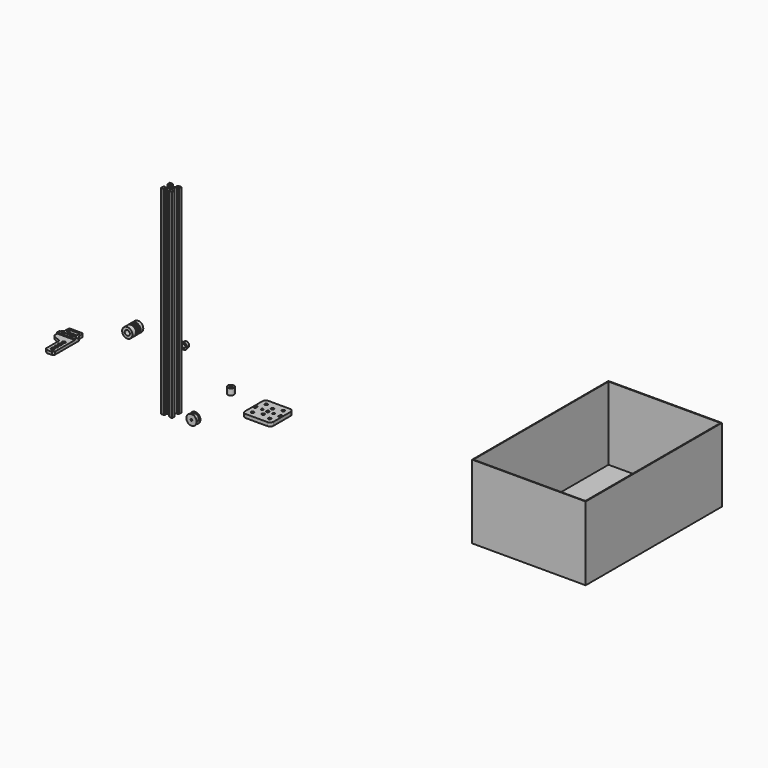
from build123d import *

# Parameters (mm, degrees)
F0_R         = 5.5
F0_R_2       = 2.5
F1_DEPTH     = 11
F2_R         = 2.51
F2_R_2       = 2
F2_W         = 2.75
F2_H         = 6.7
F3_DEPTH     = 6.35
F8_R         = 1.5
F8_R_2       = 2.15
F9_DEPTH     = 5
F10_T1_DEPTH = 20.4300979278
F10_T3_DEPTH = 14.9582429798
F11_R        = 2.1
F12_DEPTH    = 2
F14_DEPTH    = 2
F16_DEPTH    = 5
F17_SIZE     = 2
F18_W        = 199.62876
F18_H        = 299.64126
F18_W_2      = 197.0495581627
F18_H_2      = 297.1284687519
F19_DEPTH    = 129.77876
F22_DEPTH    = 350
F25_DEPTH    = 1


# Not quite as in the source:
# - a fillet or chamfer that OpenCascade refuses, or shapes differently, is made with other operations: its cross-section is extruded or revolved along the edge and cut away or added


with BuildPart() as f1:
    # F0 (on Top) → F1 (new body)
    with BuildSketch(Plane.XY):
        with Locations((46.5984568, 59.2390596867)):
            Circle(F0_R)
        with Locations((46.5984568, 59.2390596867)):
            Circle(F0_R_2, mode=Mode.SUBTRACT)
    extrude(amount=F1_DEPTH)


with BuildPart() as f3:
    # F2 (on Top) → F3 (new body)
    with BuildSketch(Plane.XY):
        with BuildLine():
            Line((145.757446865, 65.371271316), (108.097446865, 65.371271316))
            ThreePointArc((108.097446865, 65.371271316), (103.7345980251, 63.5641201559), (101.927446865, 59.201271316))
            Line((101.927446865, 59.201271316), (101.927446865, 43.721271316))
            Line((101.927446865, 43.721271316), (104.677446865, 43.721271316))
            Line((104.677446865, 43.721271316), (107.177446865, 43.721271316))
            Line((107.177446865, 43.721271316), (107.177446865, 40.371271316))
            Line((107.177446865, 40.371271316), (107.177446865, 37.021271316))
            Line((107.177446865, 37.021271316), (104.677446865, 37.021271316))
            Line((104.677446865, 37.021271316), (101.927446865, 37.021271316))
            Line((101.927446865, 37.021271316), (101.927446865, 21.541271316))
            ThreePointArc((101.927446865, 21.541271316), (103.7345980251, 17.178422476), (108.097446865, 15.371271316))
            Line((108.097446865, 15.371271316), (145.757446865, 15.371271316))
            ThreePointArc((145.757446865, 15.371271316), (150.1202957049, 17.178422476), (151.927446865, 21.541271316))
            Line((151.927446865, 21.541271316), (151.927446865, 37.021271316))
            Line((151.927446865, 37.021271316), (149.177446865, 37.021271316))
            Line((149.177446865, 37.021271316), (146.677446865, 37.021271316))
            Line((146.677446865, 37.021271316), (146.677446865, 40.371271316))
            Line((146.677446865, 40.371271316), (146.677446865, 43.721271316))
            Line((146.677446865, 43.721271316), (149.177446865, 43.721271316))
            Line((149.177446865, 43.721271316), (151.927446865, 43.721271316))
            Line((151.927446865, 43.721271316), (151.927446865, 59.201271316))
            ThreePointArc((151.927446865, 59.201271316), (150.1202957049, 63.5641201559), (145.757446865, 65.371271316))
        make_face()
        with Locations((111.927446865, 25.371271316)):
            Circle(F2_R, mode=Mode.SUBTRACT)
        with Locations((126.927446865, 30.371271316)):
            Circle(F2_R, mode=Mode.SUBTRACT)
        with Locations((116.927446865, 40.371271316)):
            Circle(F2_R_2, mode=Mode.SUBTRACT)
        with Locations((126.927446865, 40.371271316)):
            Circle(F2_R, mode=Mode.SUBTRACT)
        with Locations((141.927446865, 25.371271316)):
            Circle(F2_R, mode=Mode.SUBTRACT)
        with Locations((136.927446865, 40.371271316)):
            Circle(F2_R_2, mode=Mode.SUBTRACT)
        with Locations((126.927446865, 50.371271316)):
            Circle(F2_R, mode=Mode.SUBTRACT)
        with Locations((111.927446865, 55.371271316)):
            Circle(F2_R, mode=Mode.SUBTRACT)
        with Locations((141.927446865, 55.371271316)):
            Circle(F2_R, mode=Mode.SUBTRACT)
        Polygon((104.677446865, 43.721271316), (101.927446865, 43.721271316), (101.927446865, 40.371271316), (101.927446865, 37.021271316), (104.677446865, 37.021271316), align=None)
        with Locations((150.552446865, 40.371271316)):
            Rectangle(F2_W, F2_H)
    extrude(amount=F3_DEPTH)


with BuildPart() as f5:
    # F4 (on Top) → F5 (revolve)
    with BuildSketch(Plane.XY):
        Polygon((-173.2957138275, 117.2877326608), (-173.2957138275, 111.8661259413), (-168.7957138275, 111.8661259413), (-168.7957138275, 118.7537908554), (-172.3944602844, 117.5813526924), align=None)
        Polygon((-173.2957138275, 118.6839789152), (-173.2957138275, 117.2877326608), (-172.3944602844, 117.5813526924), (-172.3944602844, 118.9775989469), align=None)
        Polygon((-172.3944602844, 117.5813526924), (-168.7957138275, 118.7537908554), (-168.7957138275, 120.1500371099), (-172.3944602844, 118.9775989469), align=None)
        Polygon((-173.2957138275, 120.4292848706), (-173.2957138275, 118.6839789152), (-172.3944602844, 118.9775989469), (-172.3944602844, 120.7229049023), align=None)
        Polygon((-173.2957138275, 122.4000677466), (-173.2957138275, 120.4292848706), (-172.3944602844, 120.7229049023), (-172.3944602844, 122.6936877783), align=None)
        Polygon((-173.2957138275, 124.6180161834), (-173.2957138275, 122.4000677466), (-172.3944602844, 122.6936877783), (-172.3944602844, 124.911636215), align=None)
        Polygon((-172.3944602844, 122.6936877783), (-172.3944602844, 120.7229049023), (-168.7957138275, 121.8953430653), (-168.7957138275, 123.8661259413), align=None)
        Polygon((-173.2957138275, 126.642562449), (-173.2957138275, 124.6180161834), (-172.3944602844, 124.911636215), (-172.3944602844, 126.9361824806), align=None)
        Polygon((-173.2957138275, 128.4576803446), (-173.2957138275, 126.642562449), (-172.3944602844, 126.9361824806), (-172.3944602844, 128.7513003762), align=None)
        Polygon((-172.3944602844, 126.9361824806), (-172.3944602844, 124.911636215), (-168.7957138275, 126.084074378), (-168.7957138275, 128.1086206436), align=None)
        Polygon((-173.2957138275, 135.8661259413), (-173.2957138275, 128.4576803446), (-172.3944602844, 128.7513003762), (-168.7957138275, 129.9237385392), (-168.7957138275, 135.8661259413), align=None)
    revolve(axis=Axis((-177.7957138275, 123.8661259413, 0), (0, -1, 0)))


with BuildPart() as f7:
    # F6 (on Top) → F7 (revolve)
    with BuildSketch(Plane.XY):
        Polygon((-87.7572548389, 130.547894001), (-87.7572548389, 135.547894001), (-89.7572548389, 135.547894001), (-89.7572548389, 129.547894001), (-87.7572548389, 129.547894001), (-86.7572548389, 129.547894001), (-86.7572548389, 130.547894001), align=None)
    revolve(axis=Axis((-92.7572548389, 132.547894001, 0), (0, 1, 0)))


with BuildPart() as f9:
    # F8 (on Top) → F9 (new body)
    with BuildSketch(Plane.XY):
        Polygon((-214.5679742098, 55.1759666684), (-245.5969005823, 55.1759666684), (-245.5969005823, 35.1759666684), (-230.082437396, 27.7415521548), (-230.082437396, -4.2584478452), (-214.5679742098, -4.2584478452), align=None)
        with Locations((-222.3252058029, 3.7415521548)):
            Circle(F8_R, mode=Mode.SUBTRACT)
        with Locations((-222.3252058029, 11.7415521548)):
            Circle(F8_R, mode=Mode.SUBTRACT)
        with Locations((-222.3252058029, 19.7415521548)):
            Circle(F8_R, mode=Mode.SUBTRACT)
        with Locations((-237.582437396, 45.1759666684)):
            Circle(F8_R_2, mode=Mode.SUBTRACT)
        with Locations((-222.3252058029, 27.7415521548)):
            Circle(F8_R, mode=Mode.SUBTRACT)
        with Locations((-222.582437396, 45.1759666684)):
            Circle(F8_R_2, mode=Mode.SUBTRACT)
    extrude(amount=F9_DEPTH)

    # F10: chamfer of 3 on 5 edges, made by hand

    # F10_s2 → F10_t1 (cut)
    with BuildSketch(Plane.XY.offset(-7.7150489639)):
        Polygon((-230.082437396, -1.2584478452), (-227.082437396, -4.2584478452), (-230.082437396, -4.2584478452), align=None)
        Polygon((-214.5679742098, -1.2584478452), (-217.5679742098, -4.2584478452), (-214.5679742098, -4.2584478452), align=None)
        Polygon((-214.5679742098, 52.1759666684), (-217.5679742098, 55.1759666684), (-214.5679742098, 55.1759666684), align=None)
        Polygon((-242.5969005823, 55.1759666684), (-245.5969005823, 52.1759666684), (-245.5969005823, 55.1759666684), align=None)
    extrude(amount=F10_T1_DEPTH, mode=Mode.SUBTRACT)

    # F10_s4 → F10_t3 (cut)
    with BuildSketch(Plane.XY.offset(-4.9791214899)):
        Polygon((-245.5969005823, 37.0650434915), (-243.893317979, 34.3596226493), (-245.5969005823, 35.1759666684), align=None)
    extrude(amount=F10_T3_DEPTH, mode=Mode.SUBTRACT)

    # F11 (on face) → F12 (join)
    with BuildSketch(Plane.XY.offset(5)):
        Polygon((-214.5679742098, 47.6663634181), (-245.5969005823, 47.6663634181), (-245.5969005823, 42.543885321), (-214.5679742098, 42.543885321), (-214.5679742098, 44.6205050799), align=None)
        with Locations((-237.582437396, 45.1759666684)):
            Circle(F11_R, mode=Mode.SUBTRACT)
        with Locations((-222.582437396, 45.1759666684)):
            Circle(F11_R, mode=Mode.SUBTRACT)
    extrude(amount=F12_DEPTH)

    # F13 (on face) → F14 (cut)
    with BuildSketch(Plane.XY.offset(5)):
        Polygon((-220.6352813427, 24.9176974633), (-219.0347136734, 27.7931423221), (-220.7246381336, 30.6169970136), (-224.0151302631, 30.5654068464), (-225.6156979325, 27.6899619876), (-223.9257734723, 24.8661072961), align=None)
        Polygon((-220.6507124224, 16.9085198714), (-219.0344811855, 19.7751898191), (-220.708974566, 22.6082221025), (-223.9996991834, 22.5745844382), (-225.6159304203, 19.7079144906), (-223.9414370398, 16.8748822072), align=None)
        Polygon((-224.0115355835, 8.9155493468), (-220.7209804703, 8.8681463217), (-219.0346506897, 11.6941491297), (-220.6388760223, 14.5675549629), (-223.9294311356, 14.614957988), (-225.6157609161, 11.78895518), align=None)
        Polygon((-220.7013410379, 0.8791994119), (-219.0344032304, 3.7166839222), (-220.6582679954, 6.5790366651), (-223.9490705679, 6.6039048978), (-225.6160083754, 3.7664203875), (-223.9921436104, 0.9040676446), align=None)
    extrude(amount=-F14_DEPTH, mode=Mode.SUBTRACT)

    # F15 (on face) → F16 (join)
    with BuildSketch(Plane(origin=(0, 0, 0), x_dir=(1, 0, 0), z_dir=(0, 0, -1))):
        Polygon((-239.0969005823, -55.1759666684), (-242.5969005823, -55.1759666684), (-242.5969005823, -61.6759666684), (-242.5969005823, -65.1759666684), (-217.5679742098, -65.1759666684), (-217.5679742098, -61.6759666684), (-217.5679742098, -55.1759666684), (-221.0679742098, -55.1759666684), (-221.0679742098, -61.6759666684), (-239.0969005823, -61.6759666684), align=None)
    extrude(amount=-F16_DEPTH)

    # F17
    f17_edges = [f9.edges().sort_by_distance(p)[0] for p in [
        (-242.596901, 65.175967, 2.5),
        (-217.567974, 65.175967, 2.5),
    ]]
    chamfer(f17_edges, length=F17_SIZE)


with BuildPart() as f19:
    # F18 (on Top) → F19 (new body)
    with BuildSketch(Plane.XY):
        with Locations((683.4536053637, 68.4703121973)):
            Rectangle(F18_W, F18_H)
        with Locations((683.3373606205, 68.3378577232)):
            Rectangle(F18_W_2, F18_H_2, mode=Mode.SUBTRACT)
    extrude(amount=F19_DEPTH)

    # F18 (on Top) → F25 (join)
    with BuildSketch(Plane.XY):
        with Locations((683.3373606205, 68.3378577232)):
            Rectangle(F18_W_2, F18_H_2)
    extrude(amount=F25_DEPTH)


with BuildPart() as f22:
    # F21 (on Top) → F22 (new body)
    with BuildSketch(Plane.XY):
        with BuildLine():
            Line((13.7026741832, -27.698755829), (8.8896741832, -27.698755829))
            Line((8.8896741832, -27.698755829), (8.8896741832, -32.511755829))
            Line((8.8896741832, -32.511755829), (10.6896741832, -34.311755829))
            Line((10.6896741832, -34.311755829), (10.6896741832, -32.1693639626))
            Line((10.6896741832, -32.1693639626), (12.3597262214, -32.1693639626))
            Line((12.3597262214, -32.1693639626), (13.2443073387, -33.0539450799))
            Line((13.2443073387, -33.0539450799), (15.0491180878, -34.858755829))
            Line((15.0491180878, -34.858755829), (15.0491180878, -37.698755829))
            Line((15.0491180878, -37.698755829), (15.0491180878, -40.538755829))
            Line((15.0491180878, -40.538755829), (13.2443073387, -42.3435665781))
            Line((13.2443073387, -42.3435665781), (12.3597262214, -43.2281476955))
            Line((12.3597262214, -43.2281476955), (10.6896741832, -43.2281476955))
            Line((10.6896741832, -43.2281476955), (10.6896741832, -41.085755829))
            Line((10.6896741832, -41.085755829), (8.8896741832, -42.885755829))
            Line((8.8896741832, -42.885755829), (8.8896741832, -47.698755829))
            Line((8.8896741832, -47.698755829), (13.7026741832, -47.698755829))
            Line((13.7026741832, -47.698755829), (15.5026741832, -45.898755829))
            Line((15.5026741832, -45.898755829), (13.3602823167, -45.898755829))
            Line((13.3602823167, -45.898755829), (13.3602823167, -44.2287037908))
            Line((13.3602823167, -44.2287037908), (14.2448634341, -43.3441226735))
            Line((14.2448634341, -43.3441226735), (16.0496741832, -41.5393119244))
            Line((16.0496741832, -41.5393119244), (18.8896741832, -41.5393119244))
            Line((18.8896741832, -41.5393119244), (18.8896741832, -39.798755829))
            ThreePointArc((18.8896741832, -39.798755829), (17.4047499427, -36.2138315885), (20.9896741832, -37.698755829))
            Line((20.9896741832, -37.698755829), (22.7302302785, -37.698755829))
            Line((22.7302302785, -37.698755829), (22.7302302785, -34.858755829))
            Line((22.7302302785, -34.858755829), (24.5350410276, -33.0539450799))
            Line((24.5350410276, -33.0539450799), (25.419622145, -32.1693639626))
            Line((25.419622145, -32.1693639626), (27.0896741832, -32.1693639626))
            Line((27.0896741832, -32.1693639626), (27.0896741832, -34.311755829))
            Line((27.0896741832, -34.311755829), (28.8896741832, -32.511755829))
            Line((28.8896741832, -32.511755829), (28.8896741832, -27.698755829))
            Line((28.8896741832, -27.698755829), (24.0766741832, -27.698755829))
            Line((24.0766741832, -27.698755829), (22.2766741832, -29.498755829))
            Line((22.2766741832, -29.498755829), (24.4190660496, -29.498755829))
            Line((24.4190660496, -29.498755829), (24.4190660496, -31.1688078672))
            Line((24.4190660496, -31.1688078672), (23.5344849322, -32.0533889846))
            Line((23.5344849322, -32.0533889846), (21.7296741832, -33.8581997337))
            Line((21.7296741832, -33.8581997337), (18.8896741832, -33.8581997337))
            Line((18.8896741832, -33.8581997337), (16.0496741832, -33.8581997337))
            Line((16.0496741832, -33.8581997337), (14.2448634341, -32.0533889846))
            Line((14.2448634341, -32.0533889846), (13.3602823167, -31.1688078672))
            Line((13.3602823167, -31.1688078672), (13.3602823167, -29.498755829))
            Line((13.3602823167, -29.498755829), (15.5026741832, -29.498755829))
            Line((15.5026741832, -29.498755829), (13.7026741832, -27.698755829))
        make_face()
        with BuildLine():
            Line((22.7302302785, -40.538755829), (22.7302302785, -37.698755829))
            Line((22.7302302785, -37.698755829), (20.9896741832, -37.698755829))
            ThreePointArc((20.9896741832, -37.698755829), (20.3745984236, -39.1836800695), (18.8896741832, -39.798755829))
            Line((18.8896741832, -39.798755829), (18.8896741832, -41.5393119244))
            Line((18.8896741832, -41.5393119244), (21.7296741832, -41.5393119244))
            Line((21.7296741832, -41.5393119244), (23.5344849322, -43.3441226735))
            Line((23.5344849322, -43.3441226735), (24.4190660496, -44.2287037908))
            Line((24.4190660496, -44.2287037908), (24.4190660496, -45.898755829))
            Line((24.4190660496, -45.898755829), (22.2766741832, -45.898755829))
            Line((22.2766741832, -45.898755829), (24.0766741832, -47.698755829))
            Line((24.0766741832, -47.698755829), (28.8896741832, -47.698755829))
            Line((28.8896741832, -47.698755829), (28.8896741832, -42.885755829))
            Line((28.8896741832, -42.885755829), (27.0896741832, -41.085755829))
            Line((27.0896741832, -41.085755829), (27.0896741832, -43.2281476955))
            Line((27.0896741832, -43.2281476955), (25.419622145, -43.2281476955))
            Line((25.419622145, -43.2281476955), (24.5350410276, -42.3435665781))
            Line((24.5350410276, -42.3435665781), (22.7302302785, -40.538755829))
        make_face()
    extrude(amount=F22_DEPTH)


with BuildPart() as f24:
    # F23 (on Top) → F24 (revolve)
    with BuildSketch(Plane.XY):
        Polygon((62.0007956028, -26.8133749783), (54.5007956028, -26.8133749783), (54.5007956028, -35.4133749783), (59.5007956028, -35.4133749783), (62.0007956028, -35.4133749783), (62.0007956028, -34.9133749783), (59.5007956028, -34.9133749783), (59.5007956028, -27.3133749783), (62.0007956028, -27.3133749783), align=None)
    revolve(axis=Axis((53.0007956028, -31.1133749783, 0), (0, -1, 0)))


solid = Compound([f1.part, f3.part, f5.part, f7.part, f9.part, f19.part, f22.part, f24.part])
